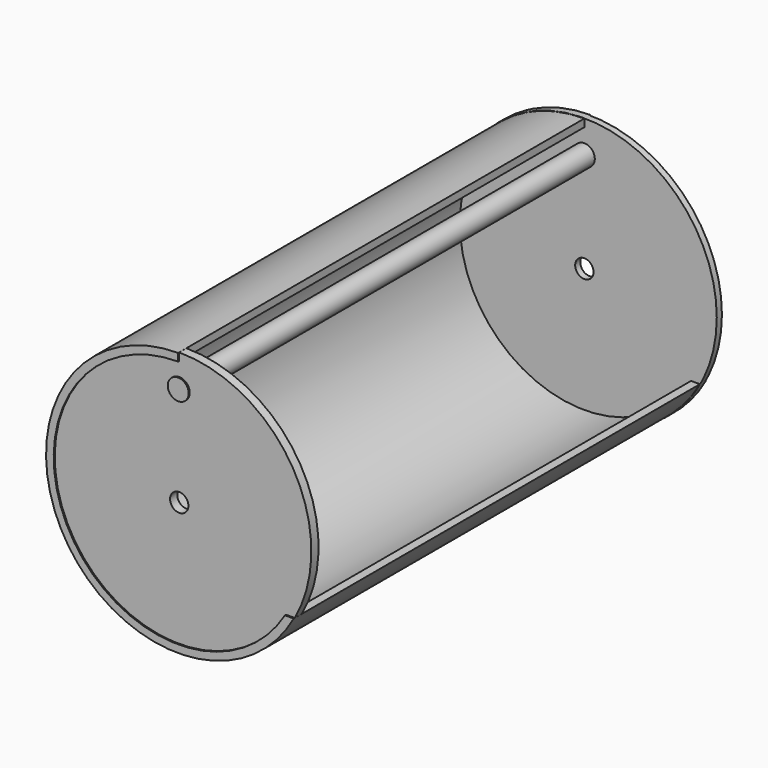
from build123d import *

# Parameters (mm, degrees)
F0_R      = 26.0530381456
F0_R_2    = 24.5437010233
F1_DEPTH  = 50.8
F2_W      = 37.793032825
F2_H      = 48.0312788859
F3_DEPTH  = 50.8
F7_START  = 48.768
F6_R      = 26.0407706564
F7_DEPTH  = 1.778
F9_START  = -49.276
F8_R      = 26.1069464333
F9_DEPTH  = 1.27
F10_R     = 2.063301756
F11_DEPTH = 50.8
F12_R     = 1.8097447332
F13_DEPTH = 50.8


# Not quite as in the source:
# - the program builds the solid bodies; features that only make, move or delete a surface that nothing else refers to are left out


with BuildPart() as f1:
    # F0 (on Front) → F1 (new body, symmetric)
    with BuildSketch(Plane.XZ):
        Circle(F0_R)
        Circle(F0_R_2, mode=Mode.SUBTRACT)
    extrude(amount=F1_DEPTH, both=True)

    # F2 (on Front) → F3 (cut, symmetric)
    with BuildSketch(Plane.XZ):
        with Locations((18.8965164125, 11.3758291118)):
            Rectangle(F2_W, F2_H)
    extrude(amount=F3_DEPTH, both=True, mode=Mode.SUBTRACT)

    # F6 (on Front) → F7 (join)
    with BuildSketch(Plane.XZ.offset(F7_START)):
        Circle(F6_R)
    extrude(amount=F7_DEPTH)

    # F8 (on Front) → F9 (join)
    with BuildSketch(Plane.XZ.offset(F9_START)):
        Circle(F8_R)
    extrude(amount=-F9_DEPTH)

    # F10 (on Front) → F11 (join, symmetric)
    with BuildSketch(Plane.XZ):
        with Locations((0, 19.7181049734)):
            Circle(F10_R)
    extrude(amount=F11_DEPTH, both=True)

    # F12 (on Front) → F13 (cut, symmetric)
    with BuildSketch(Plane.XZ):
        Circle(F12_R)
    extrude(amount=F13_DEPTH, both=True, mode=Mode.SUBTRACT)


solid = f1.part
